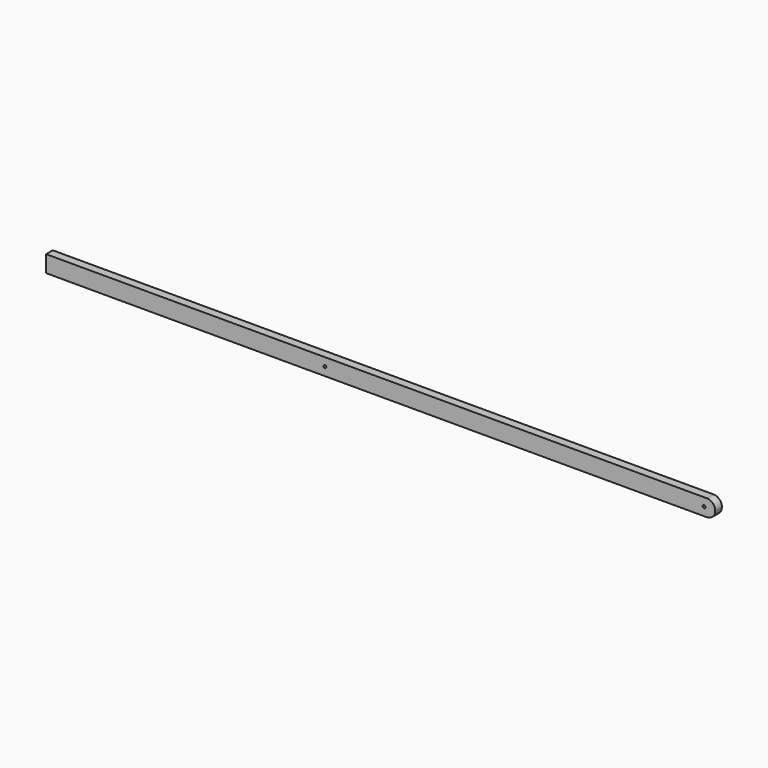
from build123d import *

# Parameters (mm, degrees)
F0_W     = 1524
F0_H     = 38.1
F0_R     = 3.175
F1_DEPTH = 19.05
F2_R     = 19.04999


# Not quite as in the source:
# - a fillet or chamfer is up to 0.001 mm smaller than in the source, because OpenCascade refuses the exact size


with BuildPart() as f1:
    # F0 (on Front) → F1 (new body)
    with BuildSketch(Plane.XZ):
        Rectangle(F0_W, F0_H)
        with Locations((-127, 0)):
            Circle(F0_R, mode=Mode.SUBTRACT)
        with Locations((736.6, 0)):
            Circle(F0_R, mode=Mode.SUBTRACT)
    extrude(amount=F1_DEPTH)

    # F2 (radius 19.05 in the source; OpenCascade refuses exactly that, so slightly less here)
    f2_edges = [f1.edges().sort_by_distance(p)[0] for p in [
        (762, -9.525, 19.05),
        (762, -9.525, -19.05),
    ]]
    fillet(f2_edges, radius=F2_R)


solid = f1.part
